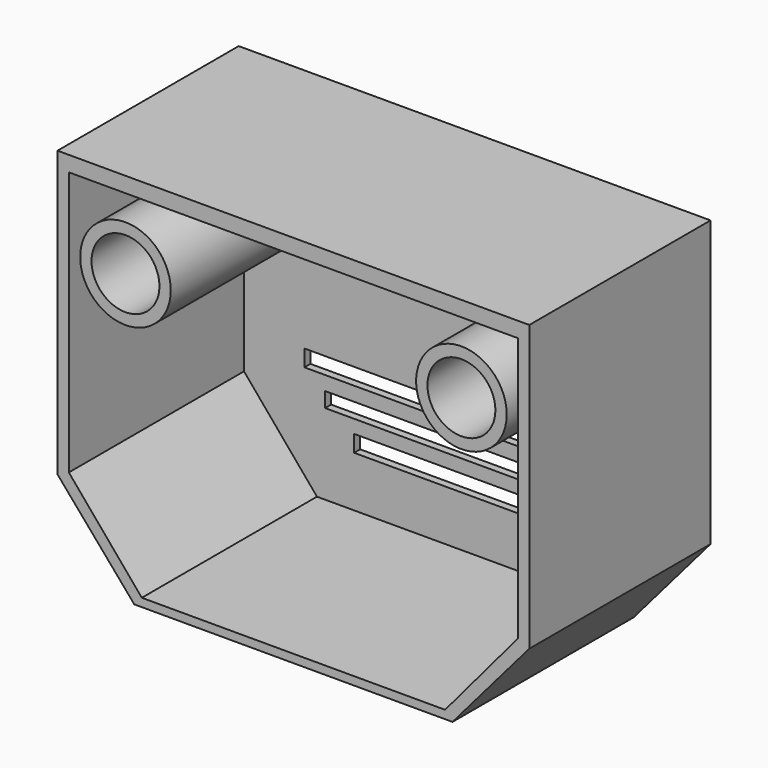
from build123d import *

# Parameters (mm, degrees)
F1_DEPTH = 76.2
F0_R     = 6.35
F0_W     = 83.9361876732
F0_H     = 5.5990750616
F0_W_2   = 100.1986385042
F0_H_2   = 5.0378413871
F0_W_3   = 111.9520328939
F0_H_3   = 5.5976028088
F0_W_4   = 15.9347772133
F0_H_4   = 5.4178200662
F0_R_2   = 15.24
F0_W_5   = 16.5721669327
F0_H_5   = 3.8243457675
F0_W_6   = 19.1217325628
F0_H_6   = 5.736514926
F0_W_7   = 17.209559679
F0_H_7   = 3.5056509078
F3_DEPTH = 2.54
F0_R_3   = 11.43
F4_DEPTH = 25.4
F5_DEPTH = 76.2


with BuildPart() as f1:
    # F0 (on Front) → F1 (new body)
    with BuildSketch(Plane.XZ):
        Polygon((99.6708340498, 77.3534489229), (-59.0791659502, 77.3534489229), (-59.0791659502, -18.5315510771), (-33.2354940474, -48.6346136725), (73.8162100315, -48.6346136725), (99.6708340498, -18.5315510771), align=None)
        Polygon((-55.2578138162, -16.7123815692), (-55.2578138162, 72.1876184308), (95.8721861838, 72.1876184308), (95.8721861838, -16.7123815692), (71.3240179544, -45.8499421496), (-30.7096455867, -45.8499421496), align=None, mode=Mode.SUBTRACT)
    extrude(amount=F1_DEPTH)

    # F0 (on Front) → F3 (join)
    with BuildSketch(Plane.XZ):
        Polygon((95.8721861838, 72.1876184308), (-55.2578138162, 72.1876184308), (-55.2578138162, -16.7123815692), (-30.7096455867, -45.8499421496), (71.3240179544, -45.8499421496), (95.8721861838, -16.7123815692), align=None)
        with Locations((23.7656522681, -25.9913175088)):
            Rectangle(F0_W, F0_H, mode=Mode.SUBTRACT)
        with Locations((22.1557993767, -16.194622498)):
            Rectangle(F0_W_2, F0_H_2, mode=Mode.SUBTRACT)
        with Locations((21.0354942828, -6.1189391417)):
            Rectangle(F0_W_3, F0_H_3, mode=Mode.SUBTRACT)
        with Locations((-5.0669364864, 45.6930417567)):
            Rectangle(F0_W_4, F0_H_4, mode=Mode.SUBTRACT)
        with Locations((-36.2078138162, 48.3655110002)):
            Circle(F0_R_2, mode=Mode.SUBTRACT)
        with Locations((-5.0669374177, 60.8310811222)):
            Rectangle(F0_W_5, F0_H_5, mode=Mode.SUBTRACT)
        with Locations((44.6495655924, 45.8523891866)):
            Rectangle(F0_W_6, F0_H_6, mode=Mode.SUBTRACT)
        with Locations((44.6495637298, 60.6717336923)):
            Rectangle(F0_W_7, F0_H_7, mode=Mode.SUBTRACT)
        with Locations((76.8221861838, 48.3655110002)):
            Circle(F0_R_2, mode=Mode.SUBTRACT)
    extrude(amount=F3_DEPTH)

    # F0 (on Front) → F4 (join)
    with BuildSketch(Plane.XZ):
        Polygon((99.6708340498, 77.3534489229), (-59.0791659502, 77.3534489229), (-59.0791659502, -18.5315510771), (-33.2354940474, -48.6346136725), (73.8162100315, -48.6346136725), (99.6708340498, -18.5315510771), align=None)
        Polygon((-55.2578138162, -16.7123815692), (-55.2578138162, 72.1876184308), (95.8721861838, 72.1876184308), (95.8721861838, -16.7123815692), (71.3240179544, -45.8499421496), (-30.7096455867, -45.8499421496), align=None, mode=Mode.SUBTRACT)
    extrude(amount=F4_DEPTH)


with BuildPart() as f1b:
    # F0 (on Front) → F1, piece 2 (new body)
    with BuildSketch(Plane.XZ):
        with Locations((-36.2078138162, 48.3655110002)):
            Circle(F0_R)
    extrude(amount=F1_DEPTH)


with BuildPart() as f3:
    # F0 (on Front) → F3, piece 2 (new body)
    with BuildSketch(Plane.XZ):
        with Locations((-36.2078138162, 48.3655110002)):
            Circle(F0_R_3)
        with Locations((-36.2078138162, 48.3655110002)):
            Circle(F0_R, mode=Mode.SUBTRACT)
    extrude(amount=F3_DEPTH)


with BuildPart() as f3b:
    # F0 (on Front) → F3, piece 3 (new body)
    with BuildSketch(Plane.XZ):
        with Locations((76.8221861838, 48.3655110002)):
            Circle(F0_R_3)
        with Locations((76.8221861838, 48.3655110002)):
            Circle(F0_R, mode=Mode.SUBTRACT)
    extrude(amount=F3_DEPTH)


with BuildPart() as f5:
    # F0 (on Front) → F5 (new body)
    with BuildSketch(Plane.XZ):
        with Locations((-36.2078138162, 48.3655110002)):
            Circle(F0_R_2)
        with Locations((-36.2078138162, 48.3655110002)):
            Circle(F0_R_3, mode=Mode.SUBTRACT)
    extrude(amount=F5_DEPTH)


with BuildPart() as f5b:
    # F0 (on Front) → F5, piece 2 (new body)
    with BuildSketch(Plane.XZ):
        with Locations((76.8221861838, 48.3655110002)):
            Circle(F0_R_2)
        with Locations((76.8221861838, 48.3655110002)):
            Circle(F0_R_3, mode=Mode.SUBTRACT)
    extrude(amount=F5_DEPTH)


solid = Compound([f1.part, f3.part, f3b.part, f5.part, f5b.part])
